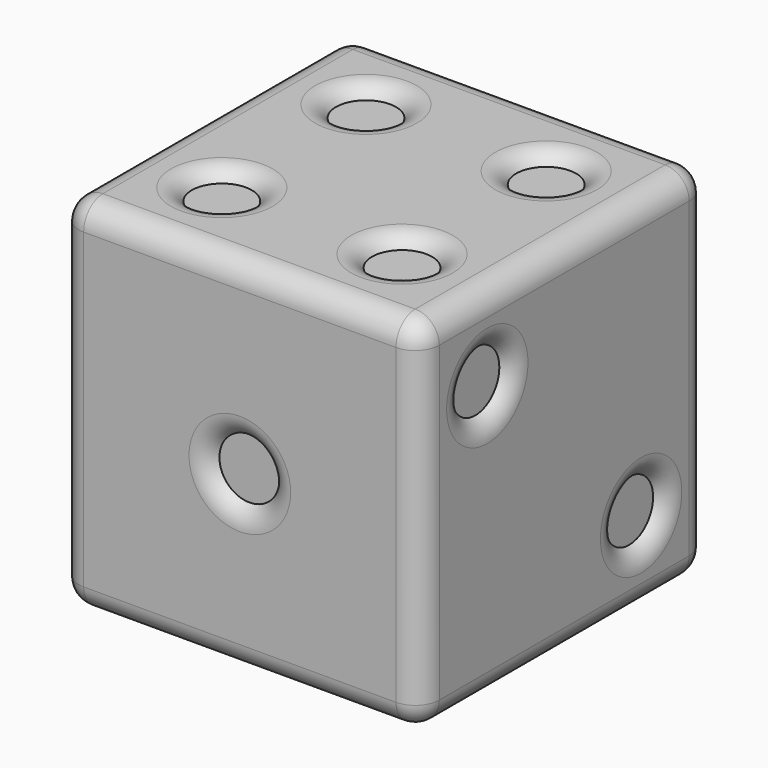
from build123d import *

# Parameters (mm, degrees)
F0_W          = 76.2
F0_H          = 76.2
F0_R          = 6.35
F1_DEPTH      = 76.2
F2_DEPTH      = 73.66
F3_R          = 6.35
F4_DEPTH      = 2.54
F5_DEPTH      = 2.54
F6_R          = 6.35
F7_DEPTH      = 2.54
F8_DEPTH      = 2.54
F9_DEPTH      = 2.54
F10_R         = 6.35
F11_DEPTH     = 2.54
F12_R         = 6.35
F13_DEPTH     = 2.54
F14_R         = 6.35
F15_DEPTH     = 2.54
F16_T1_DEPTH  = 66.04
F16_T3_DEPTH  = 66.04
F16_T5_DEPTH  = 66.04
F16_S9_W      = 5.1816
F16_S9_H      = 5.1816
F16_T10_DEPTH = 5.1816
F16_S15_W     = 5.1816
F16_S15_H     = 5.1816
F16_T16_DEPTH = 5.1816
F16_S21_W     = 5.1816
F16_S21_H     = 5.1816
F16_T22_DEPTH = 5.1816
F16_S27_W     = 5.1816
F16_S27_H     = 5.1816
F16_T28_DEPTH = 5.1816
F16_S33_W     = 5.1816
F16_S33_H     = 5.1816
F16_T34_DEPTH = 5.1816
F16_S39_W     = 5.1816
F16_S39_H     = 5.1816
F16_T40_DEPTH = 5.1816
F16_S45_W     = 5.1816
F16_S45_H     = 5.1816
F16_T46_DEPTH = 5.1816
F16_S51_W     = 5.1816
F16_S51_H     = 5.1816
F16_T52_DEPTH = 5.1816


# Not quite as in the source:
# - a fillet or chamfer that OpenCascade refuses, or shapes differently, is made with other operations: its cross-section is extruded or revolved along the edge and cut away or added


with BuildPart() as f1:
    # F0 (on Front) → F1 (new body)
    with BuildSketch(Plane.XZ):
        with Locations((-6.9278209358, 15.4253206292)):
            Rectangle(F0_W, F0_H)
        with Locations((-6.9278209358, 14.1636002809)):
            Circle(F0_R, mode=Mode.SUBTRACT)
    extrude(amount=F1_DEPTH)

    # F0 (on Front) → F2 (join)
    with BuildSketch(Plane.XZ):
        with Locations((-6.9278209358, 14.1636002809)):
            Circle(F0_R)
    extrude(amount=F2_DEPTH)

    # F3 (on face) → F4 (cut)
    with BuildSketch(Plane.YZ.offset(31.1721790642)):
        with Locations((-58.42, 35.7453206292)):
            Circle(F3_R)
    extrude(amount=-F4_DEPTH, mode=Mode.SUBTRACT)

    # F3 (on face) → F5 (cut)
    with BuildSketch(Plane.YZ.offset(31.1721790642)):
        with Locations((-17.78, -4.8946793708)):
            Circle(F3_R)
    extrude(amount=-F5_DEPTH, mode=Mode.SUBTRACT)

    # F6 (on face) → F7 (cut)
    with BuildSketch(Plane(origin=(0, 0, 0), x_dir=(-1, 0, 0), z_dir=(0, 1, 0))):
        with Locations((6.9278209358, 15.4253206292)):
            Circle(F6_R)
    extrude(amount=-F7_DEPTH, mode=Mode.SUBTRACT)

    # F6 (on face) → F8 (cut)
    with BuildSketch(Plane(origin=(0, 0, 0), x_dir=(-1, 0, 0), z_dir=(0, 1, 0))):
        with Locations((-12.1221790642, 34.4753206292)):
            Circle(F6_R)
    extrude(amount=-F8_DEPTH, mode=Mode.SUBTRACT)

    # F6 (on face) → F9 (cut)
    with BuildSketch(Plane(origin=(0, 0, 0), x_dir=(-1, 0, 0), z_dir=(0, 1, 0))):
        with Locations((25.9778209358, -3.6246793708)):
            Circle(F6_R)
    extrude(amount=-F9_DEPTH, mode=Mode.SUBTRACT)

    # F10 (on face) → F11 (cut)
    with BuildSketch(Plane.XY.offset(53.5253206292)):
        with Locations((-25.9778209358, -19.05)):
            Circle(F10_R)
        with Locations((-25.9778209358, -57.15)):
            Circle(F10_R)
        with Locations((12.1221790642, -19.05)):
            Circle(F10_R)
        with Locations((12.1221790642, -57.15)):
            Circle(F10_R)
    extrude(amount=-F11_DEPTH, mode=Mode.SUBTRACT)

    # F12 (on face) → F13 (cut)
    with BuildSketch(Plane(origin=(0, 0, -22.6746793708), x_dir=(1, 0, 0), z_dir=(0, 0, -1))):
        with Locations((-25.9778209358, 57.15)):
            Circle(F12_R)
        with Locations((-25.9778209358, 19.05)):
            Circle(F12_R)
        with Locations((-9.1552725062, 38.1)):
            Circle(F12_R)
        with Locations((12.1221790642, 57.15)):
            Circle(F12_R)
        with Locations((12.1221790642, 19.05)):
            Circle(F12_R)
    extrude(amount=-F13_DEPTH, mode=Mode.SUBTRACT)

    # F14 (on face) → F15 (cut)
    with BuildSketch(Plane(origin=(-45.0278209358, 0, 0), x_dir=(0, -1, 0), z_dir=(-1, 0, 0))):
        with Locations((19.05, -3.6246793708)):
            Circle(F14_R)
        with Locations((19.05, 15.4253206292)):
            Circle(F14_R)
        with Locations((19.05, 34.4753206292)):
            Circle(F14_R)
        with Locations((57.15, 34.4753206292)):
            Circle(F14_R)
        with Locations((57.15, 15.4253206292)):
            Circle(F14_R)
        with Locations((57.15, -3.6246793708)):
            Circle(F14_R)
    extrude(amount=-F15_DEPTH, mode=Mode.SUBTRACT)

    # F16: fillet of radius 5.08 on 33 edges, made by hand

    # F16_s2 → F16_t1 (cut)
    with BuildSketch(Plane.XY.offset(-17.5946793708)):
        with BuildLine():
            ThreePointArc((-45.0278209358, -5.08), (-43.5399233843, -1.4878975516), (-39.9478209358, 0))
            Line((-39.9478209358, 0), (-39.9478209358, 0.1016))
            Line((-39.9478209358, 0.1016), (-45.1294209358, 0.1016))
            Line((-45.1294209358, 0.1016), (-45.1294209358, -5.08))
            Line((-45.1294209358, -5.08), (-45.0278209358, -5.08))
        make_face()
        with BuildLine():
            ThreePointArc((26.0921790642, 0), (29.6842815126, -1.4878975516), (31.1721790642, -5.08))
            Line((31.1721790642, -5.08), (31.2737790642, -5.08))
            Line((31.2737790642, -5.08), (31.2737790642, 0.1016))
            Line((31.2737790642, 0.1016), (26.0921790642, 0.1016))
            Line((26.0921790642, 0.1016), (26.0921790642, 0))
        make_face()
        with BuildLine():
            ThreePointArc((26.0921790642, -76.2), (29.6842815126, -74.7121024484), (31.1721790642, -71.12))
            Line((31.1721790642, -71.12), (31.2737790642, -71.12))
            Line((31.2737790642, -71.12), (31.2737790642, -76.3016))
            Line((31.2737790642, -76.3016), (26.0921790642, -76.3016))
            Line((26.0921790642, -76.3016), (26.0921790642, -76.2))
        make_face()
        with BuildLine():
            ThreePointArc((-45.0278209358, -71.12), (-43.5399233843, -74.7121024484), (-39.9478209358, -76.2))
            Line((-39.9478209358, -76.2), (-39.9478209358, -76.3016))
            Line((-39.9478209358, -76.3016), (-45.1294209358, -76.3016))
            Line((-45.1294209358, -76.3016), (-45.1294209358, -71.12))
            Line((-45.1294209358, -71.12), (-45.0278209358, -71.12))
        make_face()
    extrude(amount=F16_T1_DEPTH, mode=Mode.SUBTRACT)

    # F16_s4 → F16_t3 (cut)
    with BuildSketch(Plane.YZ.offset(-39.9478209358)):
        with BuildLine():
            ThreePointArc((-5.08, 53.5253206292), (-1.4878975516, 52.0374230777), (0, 48.4453206292))
            Line((0, 48.4453206292), (0.1016, 48.4453206292))
            Line((0.1016, 48.4453206292), (0.1016, 53.6269206292))
            Line((0.1016, 53.6269206292), (-5.08, 53.6269206292))
            Line((-5.08, 53.6269206292), (-5.08, 53.5253206292))
        make_face()
        with BuildLine():
            ThreePointArc((0, -17.5946793708), (-1.4878975516, -21.1867818192), (-5.08, -22.6746793708))
            Line((-5.08, -22.6746793708), (-5.08, -22.7762793708))
            Line((-5.08, -22.7762793708), (0.1016, -22.7762793708))
            Line((0.1016, -22.7762793708), (0.1016, -17.5946793708))
            Line((0.1016, -17.5946793708), (0, -17.5946793708))
        make_face()
        with BuildLine():
            ThreePointArc((-71.12, 53.5253206292), (-74.7121024484, 52.0374230777), (-76.2, 48.4453206292))
            Line((-76.2, 48.4453206292), (-76.3016, 48.4453206292))
            Line((-76.3016, 48.4453206292), (-76.3016, 53.6269206292))
            Line((-76.3016, 53.6269206292), (-71.12, 53.6269206292))
            Line((-71.12, 53.6269206292), (-71.12, 53.5253206292))
        make_face()
        with BuildLine():
            ThreePointArc((-76.2, -17.5946793708), (-74.7121024484, -21.1867818192), (-71.12, -22.6746793708))
            Line((-71.12, -22.6746793708), (-71.12, -22.7762793708))
            Line((-71.12, -22.7762793708), (-76.3016, -22.7762793708))
            Line((-76.3016, -22.7762793708), (-76.3016, -17.5946793708))
            Line((-76.3016, -17.5946793708), (-76.2, -17.5946793708))
        make_face()
    extrude(amount=F16_T3_DEPTH, mode=Mode.SUBTRACT)

    # F16_s6 → F16_t5 (cut)
    with BuildSketch(Plane.XZ.offset(5.08)):
        with BuildLine():
            ThreePointArc((26.0921790642, -22.6746793708), (29.6842815126, -21.1867818192), (31.1721790642, -17.5946793708))
            Line((31.1721790642, -17.5946793708), (31.2737790642, -17.5946793708))
            Line((31.2737790642, -17.5946793708), (31.2737790642, -22.7762793708))
            Line((31.2737790642, -22.7762793708), (26.0921790642, -22.7762793708))
            Line((26.0921790642, -22.7762793708), (26.0921790642, -22.6746793708))
        make_face()
        with BuildLine():
            ThreePointArc((26.0921790642, 53.5253206292), (29.6842815126, 52.0374230777), (31.1721790642, 48.4453206292))
            Line((31.1721790642, 48.4453206292), (31.2737790642, 48.4453206292))
            Line((31.2737790642, 48.4453206292), (31.2737790642, 53.6269206292))
            Line((31.2737790642, 53.6269206292), (26.0921790642, 53.6269206292))
            Line((26.0921790642, 53.6269206292), (26.0921790642, 53.5253206292))
        make_face()
        with BuildLine():
            ThreePointArc((-45.0278209358, 48.4453206292), (-43.5399233843, 52.0374230777), (-39.9478209358, 53.5253206292))
            Line((-39.9478209358, 53.5253206292), (-39.9478209358, 53.6269206292))
            Line((-39.9478209358, 53.6269206292), (-45.1294209358, 53.6269206292))
            Line((-45.1294209358, 53.6269206292), (-45.1294209358, 48.4453206292))
            Line((-45.1294209358, 48.4453206292), (-45.0278209358, 48.4453206292))
        make_face()
        with BuildLine():
            ThreePointArc((-45.0278209358, -17.5946793708), (-43.5399233843, -21.1867818192), (-39.9478209358, -22.6746793708))
            Line((-39.9478209358, -22.6746793708), (-39.9478209358, -22.7762793708))
            Line((-39.9478209358, -22.7762793708), (-45.1294209358, -22.7762793708))
            Line((-45.1294209358, -22.7762793708), (-45.1294209358, -17.5946793708))
            Line((-45.1294209358, -17.5946793708), (-45.0278209358, -17.5946793708))
        make_face()
    extrude(amount=F16_T5_DEPTH, mode=Mode.SUBTRACT)


with BuildPart() as f16_tool8:
    # F16_s9 → F16_t10 (new body)
    with BuildSketch(Plane.YZ.offset(-39.9478209358)):
        with Locations((-2.4892, 51.0361206292)):
            Rectangle(F16_S9_W, F16_S9_H)
    extrude(amount=-F16_T10_DEPTH)

    # F16_s11 → F16_t12 (revolve, cut)
    with BuildSketch(Plane(origin=(-39.9478209358, -5.08, 48.4453206292), x_dir=(0, -0.7071067812, -0.7071067812), z_dir=(0, 0.7071067812, -0.7071067812))):
        with BuildLine():
            ThreePointArc((0, -5.08), (5.08, 0), (0, 5.08))
            Line((0, 5.08), (0, -5.08))
        make_face()
    revolve(axis=Axis((-39.9478209358, -5.08, 48.4453206292), (-1, 0, 0)), mode=Mode.SUBTRACT)


with BuildPart() as f1_1:
    add(f1.part)

    # F16_t7: cut F16_tool8
    add(f16_tool8.part, mode=Mode.SUBTRACT)


with BuildPart() as f16_tool14:
    # F16_s15 → F16_t16 (new body)
    with BuildSketch(Plane.YZ.offset(-39.9478209358)):
        with Locations((-2.4892, -20.1854793708)):
            Rectangle(F16_S15_W, F16_S15_H)
    extrude(amount=-F16_T16_DEPTH)

    # F16_s17 → F16_t18 (revolve, cut)
    with BuildSketch(Plane(origin=(-39.9478209358, -5.08, -17.5946793708), x_dir=(0, -0.7071067812, 0.7071067812), z_dir=(0, -0.7071067812, -0.7071067812))):
        with BuildLine():
            ThreePointArc((0, -5.08), (5.08, 0), (0, 5.08))
            Line((0, 5.08), (0, -5.08))
        make_face()
    revolve(axis=Axis((-39.9478209358, -5.08, -17.5946793708), (-1, 0, 0)), mode=Mode.SUBTRACT)


with BuildPart() as f1_2:
    add(f1_1.part)

    # F16_t13: cut F16_tool14
    add(f16_tool14.part, mode=Mode.SUBTRACT)


with BuildPart() as f16_tool20:
    # F16_s21 → F16_t22 (new body)
    with BuildSketch(Plane.XY.offset(48.4453206292)):
        with Locations((28.6829790642, -2.4892)):
            Rectangle(F16_S21_W, F16_S21_H)
    extrude(amount=F16_T22_DEPTH)

    # F16_s23 → F16_t24 (revolve, cut)
    with BuildSketch(Plane(origin=(26.0921790642, -5.08, 48.4453206292), x_dir=(-0.7071067812, -0.7071067812, 0), z_dir=(-0.7071067812, 0.7071067812, 0))):
        with BuildLine():
            ThreePointArc((0, -5.08), (5.08, 0), (0, 5.08))
            Line((0, 5.08), (0, -5.08))
        make_face()
    revolve(axis=Axis((26.0921790642, -5.08, 48.4453206292), (0, 0, 1)), mode=Mode.SUBTRACT)


with BuildPart() as f1_3:
    add(f1_2.part)

    # F16_t19: cut F16_tool20
    add(f16_tool20.part, mode=Mode.SUBTRACT)


with BuildPart() as f16_tool26:
    # F16_s27 → F16_t28 (new body)
    with BuildSketch(Plane.XZ.offset(5.08)):
        with Locations((28.6829790642, -20.1854793708)):
            Rectangle(F16_S27_W, F16_S27_H)
    extrude(amount=-F16_T28_DEPTH)

    # F16_s29 → F16_t30 (revolve, cut)
    with BuildSketch(Plane(origin=(26.0921790642, -5.08, -17.5946793708), x_dir=(-0.7071067812, 0, 0.7071067812), z_dir=(-0.7071067812, 0, -0.7071067812))):
        with BuildLine():
            ThreePointArc((0, -5.08), (5.08, 0), (0, 5.08))
            Line((0, 5.08), (0, -5.08))
        make_face()
    revolve(axis=Axis((26.0921790642, -5.08, -17.5946793708), (0, 1, 0)), mode=Mode.SUBTRACT)


with BuildPart() as f1_4:
    add(f1_3.part)

    # F16_t25: cut F16_tool26
    add(f16_tool26.part, mode=Mode.SUBTRACT)


with BuildPart() as f16_tool32:
    # F16_s33 → F16_t34 (new body)
    with BuildSketch(Plane.XZ.offset(71.12)):
        with Locations((28.6829790642, -20.1854793708)):
            Rectangle(F16_S33_W, F16_S33_H)
    extrude(amount=F16_T34_DEPTH)

    # F16_s35 → F16_t36 (revolve, cut)
    with BuildSketch(Plane(origin=(26.0921790642, -71.12, -17.5946793708), x_dir=(-0.7071067812, 0, 0.7071067812), z_dir=(0.7071067812, 0, 0.7071067812))):
        with BuildLine():
            ThreePointArc((0, -5.08), (5.08, 0), (0, 5.08))
            Line((0, 5.08), (0, -5.08))
        make_face()
    revolve(axis=Axis((26.0921790642, -71.12, -17.5946793708), (0, -1, 0)), mode=Mode.SUBTRACT)


with BuildPart() as f1_5:
    add(f1_4.part)

    # F16_t31: cut F16_tool32
    add(f16_tool32.part, mode=Mode.SUBTRACT)


with BuildPart() as f16_tool38:
    # F16_s39 → F16_t40 (new body)
    with BuildSketch(Plane.YZ.offset(26.0921790642)):
        with Locations((-73.7108, 51.0361206292)):
            Rectangle(F16_S39_W, F16_S39_H)
    extrude(amount=F16_T40_DEPTH)

    # F16_s41 → F16_t42 (revolve, cut)
    with BuildSketch(Plane(origin=(26.0921790642, -71.12, 48.4453206292), x_dir=(0, 0.7071067812, -0.7071067812), z_dir=(0, -0.7071067812, -0.7071067812))):
        with BuildLine():
            ThreePointArc((0, -5.08), (5.08, 0), (0, 5.08))
            Line((0, 5.08), (0, -5.08))
        make_face()
    revolve(axis=Axis((26.0921790642, -71.12, 48.4453206292), (1, 0, 0)), mode=Mode.SUBTRACT)


with BuildPart() as f1_6:
    add(f1_5.part)

    # F16_t37: cut F16_tool38
    add(f16_tool38.part, mode=Mode.SUBTRACT)


with BuildPart() as f16_tool44:
    # F16_s45 → F16_t46 (new body)
    with BuildSketch(Plane.YZ.offset(-39.9478209358)):
        with Locations((-73.7108, 51.0361206292)):
            Rectangle(F16_S45_W, F16_S45_H)
    extrude(amount=-F16_T46_DEPTH)

    # F16_s47 → F16_t48 (revolve, cut)
    with BuildSketch(Plane(origin=(-39.9478209358, -71.12, 48.4453206292), x_dir=(0, 0.7071067812, -0.7071067812), z_dir=(0, 0.7071067812, 0.7071067812))):
        with BuildLine():
            ThreePointArc((0, -5.08), (5.08, 0), (0, 5.08))
            Line((0, 5.08), (0, -5.08))
        make_face()
    revolve(axis=Axis((-39.9478209358, -71.12, 48.4453206292), (-1, 0, 0)), mode=Mode.SUBTRACT)


with BuildPart() as f1_7:
    add(f1_6.part)

    # F16_t43: cut F16_tool44
    add(f16_tool44.part, mode=Mode.SUBTRACT)


with BuildPart() as f16_tool50:
    # F16_s51 → F16_t52 (new body)
    with BuildSketch(Plane.YZ.offset(-39.9478209358)):
        with Locations((-73.7108, -20.1854793708)):
            Rectangle(F16_S51_W, F16_S51_H)
    extrude(amount=-F16_T52_DEPTH)

    # F16_s53 → F16_t54 (revolve, cut)
    with BuildSketch(Plane(origin=(-39.9478209358, -71.12, -17.5946793708), x_dir=(0, 0.7071067812, 0.7071067812), z_dir=(0, -0.7071067812, 0.7071067812))):
        with BuildLine():
            ThreePointArc((0, -5.08), (5.08, 0), (0, 5.08))
            Line((0, 5.08), (0, -5.08))
        make_face()
    revolve(axis=Axis((-39.9478209358, -71.12, -17.5946793708), (-1, 0, 0)), mode=Mode.SUBTRACT)


with BuildPart() as f1_8:
    add(f1_7.part)

    # F16_t49: cut F16_tool50
    add(f16_tool50.part, mode=Mode.SUBTRACT)

    # F16_s55 → F16_t56 (revolve, cut)
    with BuildSketch(Plane.XY.offset(-3.6246793708)):
        with BuildLine():
            ThreePointArc((-36.7272299871, 0), (-34.1872299871, -0.6805909488), (-32.3278209358, -2.54))
            Line((-32.3278209358, -2.54), (-32.2398327548, -2.4892))
            ThreePointArc((-32.2398327548, -2.4892), (-32.2262209358, -1.27), (-32.2262209358, 0))
            Line((-32.2262209358, 0), (-32.3278209358, 0.1016))
            Line((-32.3278209358, 0.1016), (-36.7272299871, 0.1016))
            Line((-36.7272299871, 0.1016), (-36.7272299871, 0))
        make_face()
    revolve(axis=Axis((-25.9778209358, 0, -3.6246793708), (0, 1, 0)), mode=Mode.SUBTRACT)

    # F16_s57 → F16_t58 (revolve, cut)
    with BuildSketch(Plane.XY.offset(15.4253206292)):
        with BuildLine():
            ThreePointArc((-17.6772299871, 0), (-15.1372299871, -0.6805909488), (-13.2778209358, -2.54))
            Line((-13.2778209358, -2.54), (-13.1898327548, -2.4892))
            ThreePointArc((-13.1898327548, -2.4892), (-13.1762209358, -1.27), (-13.1762209358, 0))
            Line((-13.1762209358, 0), (-13.2778209358, 0.1016))
            Line((-13.2778209358, 0.1016), (-17.6772299871, 0.1016))
            Line((-17.6772299871, 0.1016), (-17.6772299871, 0))
        make_face()
    revolve(axis=Axis((-6.9278209358, 0, 15.4253206292), (0, 1, 0)), mode=Mode.SUBTRACT)

    # F16_s59 → F16_t60 (revolve, cut)
    with BuildSketch(Plane.XY.offset(34.4753206292)):
        with BuildLine():
            ThreePointArc((1.3727700129, 0), (3.9127700129, -0.6805909488), (5.7721790642, -2.54))
            Line((5.7721790642, -2.54), (5.8601672452, -2.4892))
            ThreePointArc((5.8601672452, -2.4892), (5.8737790642, -1.27), (5.8737790642, 0))
            Line((5.8737790642, 0), (5.7721790642, 0.1016))
            Line((5.7721790642, 0.1016), (1.3727700129, 0.1016))
            Line((1.3727700129, 0.1016), (1.3727700129, 0))
        make_face()
    revolve(axis=Axis((12.1221790642, 0, 34.4753206292), (0, 1, 0)), mode=Mode.SUBTRACT)

    # F16_s61 → F16_t62 (revolve, cut)
    with BuildSketch(Plane.XY.offset(35.7453206292)):
        with BuildLine():
            ThreePointArc((31.1721790642, -47.6705909488), (30.4915881154, -50.2105909488), (28.6321790642, -52.07))
            Line((28.6321790642, -52.07), (28.6829790642, -52.157988181))
            ThreePointArc((28.6829790642, -52.157988181), (29.9021790642, -52.1716), (31.1721790642, -52.1716))
            Line((31.1721790642, -52.1716), (31.2737790642, -52.07))
            Line((31.2737790642, -52.07), (31.2737790642, -47.6705909488))
            Line((31.2737790642, -47.6705909488), (31.1721790642, -47.6705909488))
        make_face()
    revolve(axis=Axis((31.1721790642, -58.42, 35.7453206292), (1, 0, 0)), mode=Mode.SUBTRACT)

    # F16_s63 → F16_t64 (revolve, cut)
    with BuildSketch(Plane.XY.offset(-4.8946793708)):
        with BuildLine():
            ThreePointArc((31.1721790642, -7.0305909488), (30.4915881154, -9.5705909488), (28.6321790642, -11.43))
            Line((28.6321790642, -11.43), (28.6829790642, -11.517988181))
            ThreePointArc((28.6829790642, -11.517988181), (29.9021790642, -11.5316), (31.1721790642, -11.5316))
            Line((31.1721790642, -11.5316), (31.2737790642, -11.43))
            Line((31.2737790642, -11.43), (31.2737790642, -7.0305909488))
            Line((31.2737790642, -7.0305909488), (31.1721790642, -7.0305909488))
        make_face()
    revolve(axis=Axis((31.1721790642, -17.78, -4.8946793708), (1, 0, 0)), mode=Mode.SUBTRACT)

    # F16_s65 → F16_t66 (revolve, cut)
    with BuildSketch(Plane.XZ.offset(57.15)):
        with BuildLine():
            ThreePointArc((22.8715881154, 53.5253206292), (20.3315881154, 52.8447296805), (18.4721790642, 50.9853206292))
            Line((18.4721790642, 50.9853206292), (18.3841908831, 51.0361206292))
            ThreePointArc((18.3841908831, 51.0361206292), (18.3705790642, 52.2553206292), (18.3705790642, 53.5253206292))
            Line((18.3705790642, 53.5253206292), (18.4721790642, 53.6269206292))
            Line((18.4721790642, 53.6269206292), (22.8715881154, 53.6269206292))
            Line((22.8715881154, 53.6269206292), (22.8715881154, 53.5253206292))
        make_face()
    revolve(axis=Axis((12.1221790642, -57.15, 53.5253206292), (0, 0, 1)), mode=Mode.SUBTRACT)

    # F16_s67 → F16_t68 (revolve, cut)
    with BuildSketch(Plane.XZ.offset(57.15)):
        with BuildLine():
            ThreePointArc((-15.2284118846, 53.5253206292), (-17.7684118846, 52.8447296805), (-19.6278209358, 50.9853206292))
            Line((-19.6278209358, 50.9853206292), (-19.7158091169, 51.0361206292))
            ThreePointArc((-19.7158091169, 51.0361206292), (-19.7294209358, 52.2553206292), (-19.7294209358, 53.5253206292))
            Line((-19.7294209358, 53.5253206292), (-19.6278209358, 53.6269206292))
            Line((-19.6278209358, 53.6269206292), (-15.2284118846, 53.6269206292))
            Line((-15.2284118846, 53.6269206292), (-15.2284118846, 53.5253206292))
        make_face()
    revolve(axis=Axis((-25.9778209358, -57.15, 53.5253206292), (0, 0, 1)), mode=Mode.SUBTRACT)

    # F16_s69 → F16_t70 (revolve, cut)
    with BuildSketch(Plane.XZ.offset(19.05)):
        with BuildLine():
            ThreePointArc((22.8715881154, 53.5253206292), (20.3315881154, 52.8447296805), (18.4721790642, 50.9853206292))
            Line((18.4721790642, 50.9853206292), (18.3841908831, 51.0361206292))
            ThreePointArc((18.3841908831, 51.0361206292), (18.3705790642, 52.2553206292), (18.3705790642, 53.5253206292))
            Line((18.3705790642, 53.5253206292), (18.4721790642, 53.6269206292))
            Line((18.4721790642, 53.6269206292), (22.8715881154, 53.6269206292))
            Line((22.8715881154, 53.6269206292), (22.8715881154, 53.5253206292))
        make_face()
    revolve(axis=Axis((12.1221790642, -19.05, 53.5253206292), (0, 0, 1)), mode=Mode.SUBTRACT)

    # F16_s71 → F16_t72 (revolve, cut)
    with BuildSketch(Plane.XZ.offset(19.05)):
        with BuildLine():
            ThreePointArc((-15.2284118846, 53.5253206292), (-17.7684118846, 52.8447296805), (-19.6278209358, 50.9853206292))
            Line((-19.6278209358, 50.9853206292), (-19.7158091169, 51.0361206292))
            ThreePointArc((-19.7158091169, 51.0361206292), (-19.7294209358, 52.2553206292), (-19.7294209358, 53.5253206292))
            Line((-19.7294209358, 53.5253206292), (-19.6278209358, 53.6269206292))
            Line((-19.6278209358, 53.6269206292), (-15.2284118846, 53.6269206292))
            Line((-15.2284118846, 53.6269206292), (-15.2284118846, 53.5253206292))
        make_face()
    revolve(axis=Axis((-25.9778209358, -19.05, 53.5253206292), (0, 0, 1)), mode=Mode.SUBTRACT)

    # F16_s73 → F16_t74 (revolve, cut)
    with BuildSketch(Plane.XY.offset(34.4753206292)):
        with BuildLine():
            ThreePointArc((-45.0278209358, -67.8994090512), (-44.3472299871, -65.3594090512), (-42.4878209358, -63.5))
            Line((-42.4878209358, -63.5), (-42.5386209358, -63.412011819))
            ThreePointArc((-42.5386209358, -63.412011819), (-43.7578209358, -63.3984), (-45.0278209358, -63.3984))
            Line((-45.0278209358, -63.3984), (-45.1294209358, -63.5))
            Line((-45.1294209358, -63.5), (-45.1294209358, -67.8994090512))
            Line((-45.1294209358, -67.8994090512), (-45.0278209358, -67.8994090512))
        make_face()
    revolve(axis=Axis((-45.0278209358, -57.15, 34.4753206292), (-1, 0, 0)), mode=Mode.SUBTRACT)

    # F16_s75 → F16_t76 (revolve, cut)
    with BuildSketch(Plane.XY.offset(15.4253206292)):
        with BuildLine():
            ThreePointArc((-45.0278209358, -67.8994090512), (-44.3472299871, -65.3594090512), (-42.4878209358, -63.5))
            Line((-42.4878209358, -63.5), (-42.5386209358, -63.412011819))
            ThreePointArc((-42.5386209358, -63.412011819), (-43.7578209358, -63.3984), (-45.0278209358, -63.3984))
            Line((-45.0278209358, -63.3984), (-45.1294209358, -63.5))
            Line((-45.1294209358, -63.5), (-45.1294209358, -67.8994090512))
            Line((-45.1294209358, -67.8994090512), (-45.0278209358, -67.8994090512))
        make_face()
    revolve(axis=Axis((-45.0278209358, -57.15, 15.4253206292), (-1, 0, 0)), mode=Mode.SUBTRACT)

    # F16_s77 → F16_t78 (revolve, cut)
    with BuildSketch(Plane.XY.offset(-3.6246793708)):
        with BuildLine():
            ThreePointArc((-45.0278209358, -67.8994090512), (-44.3472299871, -65.3594090512), (-42.4878209358, -63.5))
            Line((-42.4878209358, -63.5), (-42.5386209358, -63.412011819))
            ThreePointArc((-42.5386209358, -63.412011819), (-43.7578209358, -63.3984), (-45.0278209358, -63.3984))
            Line((-45.0278209358, -63.3984), (-45.1294209358, -63.5))
            Line((-45.1294209358, -63.5), (-45.1294209358, -67.8994090512))
            Line((-45.1294209358, -67.8994090512), (-45.0278209358, -67.8994090512))
        make_face()
    revolve(axis=Axis((-45.0278209358, -57.15, -3.6246793708), (-1, 0, 0)), mode=Mode.SUBTRACT)

    # F16_s79 → F16_t80 (revolve, cut)
    with BuildSketch(Plane.XY.offset(34.4753206292)):
        with BuildLine():
            ThreePointArc((-45.0278209358, -29.7994090512), (-44.3472299871, -27.2594090512), (-42.4878209358, -25.4))
            Line((-42.4878209358, -25.4), (-42.5386209358, -25.312011819))
            ThreePointArc((-42.5386209358, -25.312011819), (-43.7578209358, -25.2984), (-45.0278209358, -25.2984))
            Line((-45.0278209358, -25.2984), (-45.1294209358, -25.4))
            Line((-45.1294209358, -25.4), (-45.1294209358, -29.7994090512))
            Line((-45.1294209358, -29.7994090512), (-45.0278209358, -29.7994090512))
        make_face()
    revolve(axis=Axis((-45.0278209358, -19.05, 34.4753206292), (-1, 0, 0)), mode=Mode.SUBTRACT)

    # F16_s81 → F16_t82 (revolve, cut)
    with BuildSketch(Plane.XY.offset(15.4253206292)):
        with BuildLine():
            ThreePointArc((-45.0278209358, -29.7994090512), (-44.3472299871, -27.2594090512), (-42.4878209358, -25.4))
            Line((-42.4878209358, -25.4), (-42.5386209358, -25.312011819))
            ThreePointArc((-42.5386209358, -25.312011819), (-43.7578209358, -25.2984), (-45.0278209358, -25.2984))
            Line((-45.0278209358, -25.2984), (-45.1294209358, -25.4))
            Line((-45.1294209358, -25.4), (-45.1294209358, -29.7994090512))
            Line((-45.1294209358, -29.7994090512), (-45.0278209358, -29.7994090512))
        make_face()
    revolve(axis=Axis((-45.0278209358, -19.05, 15.4253206292), (-1, 0, 0)), mode=Mode.SUBTRACT)

    # F16_s83 → F16_t84 (revolve, cut)
    with BuildSketch(Plane.XY.offset(-3.6246793708)):
        with BuildLine():
            ThreePointArc((-45.0278209358, -29.7994090512), (-44.3472299871, -27.2594090512), (-42.4878209358, -25.4))
            Line((-42.4878209358, -25.4), (-42.5386209358, -25.312011819))
            ThreePointArc((-42.5386209358, -25.312011819), (-43.7578209358, -25.2984), (-45.0278209358, -25.2984))
            Line((-45.0278209358, -25.2984), (-45.1294209358, -25.4))
            Line((-45.1294209358, -25.4), (-45.1294209358, -29.7994090512))
            Line((-45.1294209358, -29.7994090512), (-45.0278209358, -29.7994090512))
        make_face()
    revolve(axis=Axis((-45.0278209358, -19.05, -3.6246793708), (-1, 0, 0)), mode=Mode.SUBTRACT)

    # F16_s85 → F16_t86 (revolve, cut)
    with BuildSketch(Plane.XY.offset(14.1636002809)):
        with BuildLine():
            ThreePointArc((3.8215881154, -76.2), (1.2815881154, -75.5194090512), (-0.5778209358, -73.66))
            Line((-0.5778209358, -73.66), (-0.6658091169, -73.7108))
            ThreePointArc((-0.6658091169, -73.7108), (-0.6794209358, -74.93), (-0.6794209358, -76.2))
            Line((-0.6794209358, -76.2), (-0.5778209358, -76.3016))
            Line((-0.5778209358, -76.3016), (3.8215881154, -76.3016))
            Line((3.8215881154, -76.3016), (3.8215881154, -76.2))
        make_face()
    revolve(axis=Axis((-6.9278209358, -76.2, 14.1636002809), (0, -1, 0)), mode=Mode.SUBTRACT)

    # F16_s87 → F16_t88 (revolve, cut)
    with BuildSketch(Plane.XZ.offset(57.15)):
        with BuildLine():
            ThreePointArc((-15.2284118846, -22.6746793708), (-17.7684118846, -21.994088422), (-19.6278209358, -20.1346793708))
            Line((-19.6278209358, -20.1346793708), (-19.7158091169, -20.1854793708))
            ThreePointArc((-19.7158091169, -20.1854793708), (-19.7294209358, -21.4046793708), (-19.7294209358, -22.6746793708))
            Line((-19.7294209358, -22.6746793708), (-19.6278209358, -22.7762793708))
            Line((-19.6278209358, -22.7762793708), (-15.2284118846, -22.7762793708))
            Line((-15.2284118846, -22.7762793708), (-15.2284118846, -22.6746793708))
        make_face()
    revolve(axis=Axis((-25.9778209358, -57.15, -22.6746793708), (0, 0, -1)), mode=Mode.SUBTRACT)

    # F16_s89 → F16_t90 (revolve, cut)
    with BuildSketch(Plane.XZ.offset(38.1)):
        with BuildLine():
            ThreePointArc((1.594136545, -22.6746793708), (-0.945863455, -21.994088422), (-2.8052725062, -20.1346793708))
            Line((-2.8052725062, -20.1346793708), (-2.8932606872, -20.1854793708))
            ThreePointArc((-2.8932606872, -20.1854793708), (-2.9068725062, -21.4046793708), (-2.9068725062, -22.6746793708))
            Line((-2.9068725062, -22.6746793708), (-2.8052725062, -22.7762793708))
            Line((-2.8052725062, -22.7762793708), (1.594136545, -22.7762793708))
            Line((1.594136545, -22.7762793708), (1.594136545, -22.6746793708))
        make_face()
    revolve(axis=Axis((-9.1552725062, -38.1, -22.6746793708), (0, 0, -1)), mode=Mode.SUBTRACT)

    # F16_s91 → F16_t92 (revolve, cut)
    with BuildSketch(Plane.XZ.offset(57.15)):
        with BuildLine():
            ThreePointArc((22.8715881154, -22.6746793708), (20.3315881154, -21.994088422), (18.4721790642, -20.1346793708))
            Line((18.4721790642, -20.1346793708), (18.3841908831, -20.1854793708))
            ThreePointArc((18.3841908831, -20.1854793708), (18.3705790642, -21.4046793708), (18.3705790642, -22.6746793708))
            Line((18.3705790642, -22.6746793708), (18.4721790642, -22.7762793708))
            Line((18.4721790642, -22.7762793708), (22.8715881154, -22.7762793708))
            Line((22.8715881154, -22.7762793708), (22.8715881154, -22.6746793708))
        make_face()
    revolve(axis=Axis((12.1221790642, -57.15, -22.6746793708), (0, 0, -1)), mode=Mode.SUBTRACT)

    # F16_s93 → F16_t94 (revolve, cut)
    with BuildSketch(Plane.XZ.offset(19.05)):
        with BuildLine():
            ThreePointArc((-15.2284118846, -22.6746793708), (-17.7684118846, -21.994088422), (-19.6278209358, -20.1346793708))
            Line((-19.6278209358, -20.1346793708), (-19.7158091169, -20.1854793708))
            ThreePointArc((-19.7158091169, -20.1854793708), (-19.7294209358, -21.4046793708), (-19.7294209358, -22.6746793708))
            Line((-19.7294209358, -22.6746793708), (-19.6278209358, -22.7762793708))
            Line((-19.6278209358, -22.7762793708), (-15.2284118846, -22.7762793708))
            Line((-15.2284118846, -22.7762793708), (-15.2284118846, -22.6746793708))
        make_face()
    revolve(axis=Axis((-25.9778209358, -19.05, -22.6746793708), (0, 0, -1)), mode=Mode.SUBTRACT)

    # F16_s95 → F16_t96 (revolve, cut)
    with BuildSketch(Plane.XZ.offset(19.05)):
        with BuildLine():
            ThreePointArc((22.8715881154, -22.6746793708), (20.3315881154, -21.994088422), (18.4721790642, -20.1346793708))
            Line((18.4721790642, -20.1346793708), (18.3841908831, -20.1854793708))
            ThreePointArc((18.3841908831, -20.1854793708), (18.3705790642, -21.4046793708), (18.3705790642, -22.6746793708))
            Line((18.3705790642, -22.6746793708), (18.4721790642, -22.7762793708))
            Line((18.4721790642, -22.7762793708), (22.8715881154, -22.7762793708))
            Line((22.8715881154, -22.7762793708), (22.8715881154, -22.6746793708))
        make_face()
    revolve(axis=Axis((12.1221790642, -19.05, -22.6746793708), (0, 0, -1)), mode=Mode.SUBTRACT)


solid = f1_8.part
